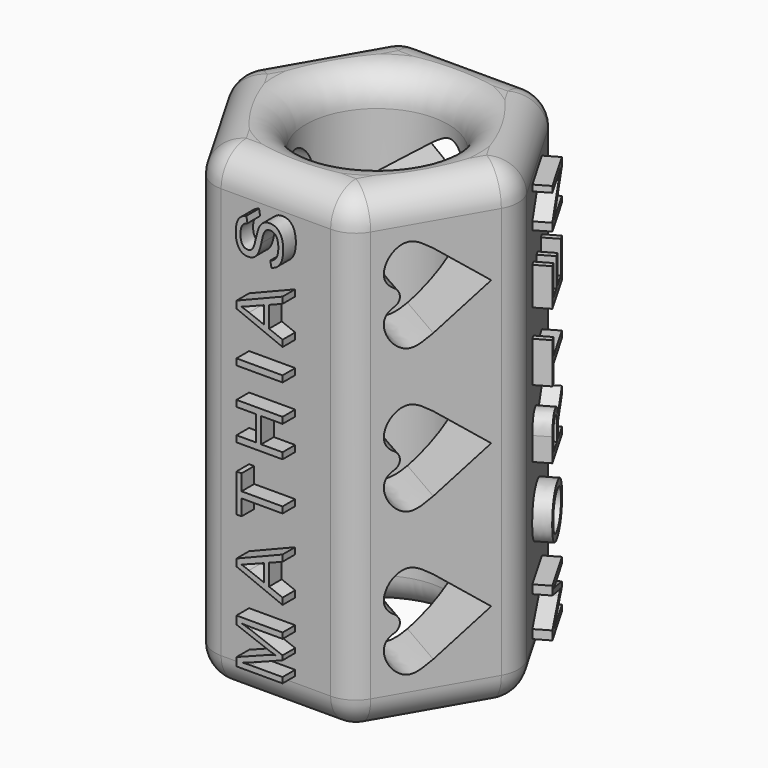
from build123d import *

# Parameters (mm, degrees)
F0_R          = 2.25
F1_DEPTH      = 15
F2_TEXT_SIZE  = 2.9915144542
F3_DEPTH      = 0.5
F4_TEXT_SIZE  = 2.2767698328
F5_DEPTH      = 0.5
F6_TEXT_SIZE  = 2.1189354387
F7_DEPTH      = 0.5
F9_DEPTH      = 5
F11_DEPTH     = 5
F13_DEPTH     = 5
F14_T1_DEPTH  = 9.6188021535
F14_T3_DEPTH  = 9.6188021535
F14_T5_DEPTH  = 9.6188021535
F14_T7_DEPTH  = 9.6188021535
F14_T9_DEPTH  = 9.6188021535
F15_T1_DEPTH  = 13
F15_T6_DEPTH  = 1
F15_T12_DEPTH = 1
F15_T18_DEPTH = 1
F15_T24_DEPTH = 1
F15_T30_DEPTH = 1
F15_T36_DEPTH = 1
F15_T42_DEPTH = 1
F15_T48_DEPTH = 1
F15_T54_DEPTH = 1
F15_T60_DEPTH = 1
F15_T66_DEPTH = 1
F15_T72_DEPTH = 1
F16_R         = 0.3


# Not quite as in the source:
# - a fillet or chamfer that OpenCascade refuses, or shapes differently, is made with other operations: its cross-section is extruded or revolved along the edge and cut away or added
# - Text() gives the source's letters only with a copy of the font that has no kerning and outlines rounded to 1/6400 em; it was checked with that copy


with BuildPart() as f1:
    # F0 (on Top) → F1 (new body)
    with BuildSketch(Plane.XY):
        Polygon((-2.3094010768, -4), (2.3094010768, -4), (4.6188021535, 0), (2.3094010768, 4), (-2.3094010768, 4), (-4.6188021535, 0), align=None)
        Circle(F0_R, mode=Mode.SUBTRACT)
    extrude(amount=F1_DEPTH)

    # F2 (on face) → F3 (join)
    with BuildSketch(Plane(origin=(-3.4641016151, 2, 0), x_dir=(-0.5, -0.8660254038, 0), z_dir=(-0.8660254038, 0.5, 0))):
        with Locations(Location((0.9215387268, 1), (0, 0, 90))):
            Text('M A R I A', F2_TEXT_SIZE, font='Arimo', text_align=(TextAlign.LEFT, TextAlign.BOTTOM))
    extrude(amount=F3_DEPTH)

    # F4 (on face) → F5 (join)
    with BuildSketch(Plane(origin=(3.4641016151, 2, 0), x_dir=(-0.5, 0.8660254038, 0), z_dir=(0.8660254038, 0.5, 0))):
        with Locations(Location((0.7773110224, 0.9308314361), (0, 0, 90))):
            Text('M O R T E N', F4_TEXT_SIZE, font='Arimo', text_align=(TextAlign.LEFT, TextAlign.BOTTOM))
    extrude(amount=F5_DEPTH)

    # F6 (on face) → F7 (join)
    with BuildSketch(Plane.XZ.offset(4)):
        with Locations(Location((0.6108914517, 1.017461665), (0, 0, 90))):
            Text('M A T H I A S', F6_TEXT_SIZE, font='Arimo', text_align=(TextAlign.LEFT, TextAlign.BOTTOM))
    extrude(amount=F7_DEPTH)

    # F8 (on face) → F9 (cut)
    with BuildSketch(Plane(origin=(-3.4641016151, -2, 0), x_dir=(0.5, -0.8660254038, 0), z_dir=(-0.8660254038, -0.5, 0))):
        with BuildLine():
            Line((0, 1.776238773), (1.5377772506, 2.9594601877))
            Line((1.5377772506, 2.9594601877), (0, 4.1426816024))
            add(Edge.make_bspline(
                [(0, 4.1426816024), (-0.2173509057, 4.2946153333), (-0.6310612999, 4.5838092683), (-1.2004435179, 4.1850955605), (-1.3756111709, 3.5968057921), (-1.1404542273, 3.2179649778), (-0.5606131931, 3.0412608869), (-0.1866981793, 2.9867018613), (0, 2.9594601877)],
                knots=[0, 0, 0, 0, 0.1874012518, 0.3567035782, 0.5239209237, 0.6616950004, 0.8310821306, 1, 1, 1, 1], degree=3))
            add(Edge.make_bspline(
                [(0, 1.776238773), (-0.2173509057, 1.6243050422), (-0.6310612999, 1.3351111071), (-1.2004435179, 1.7338248149), (-1.3756111709, 2.3221145833), (-1.1404542273, 2.7009553976), (-0.5606131931, 2.8776594885), (-0.1866981793, 2.9322185141), (0, 2.9594601877)],
                knots=[0, 0, 0, 0, 0.1874012518, 0.3567035782, 0.5239209237, 0.6616950004, 0.8310821306, 1, 1, 1, 1], degree=3))
        make_face()
        with BuildLine():
            Line((0, 6.3167785853), (1.5377772506, 7.5))
            Line((1.5377772506, 7.5), (0, 8.6832214147))
            add(Edge.make_bspline(
                [(0, 8.6832214147), (-0.2173509057, 8.8351551455), (-0.6310612999, 9.1243490806), (-1.2004435179, 8.7256353728), (-1.3756111709, 8.1373456044), (-1.1404542273, 7.7585047901), (-0.5606131931, 7.5818006992), (-0.1866981793, 7.5272416736), (0, 7.5)],
                knots=[0, 0, 0, 0, 0.1874012518, 0.3567035782, 0.5239209237, 0.6616950004, 0.8310821306, 1, 1, 1, 1], degree=3))
            add(Edge.make_bspline(
                [(0, 6.3167785853), (-0.2173509057, 6.1648448545), (-0.6310612999, 5.8756509194), (-1.2004435179, 6.2743646272), (-1.3756111709, 6.8626543956), (-1.1404542273, 7.2414952099), (-0.5606131931, 7.4181993008), (-0.1866981793, 7.4727583264), (0, 7.5)],
                knots=[0, 0, 0, 0, 0.1874012518, 0.3567035782, 0.5239209237, 0.6616950004, 0.8310821306, 1, 1, 1, 1], degree=3))
        make_face()
        with BuildLine():
            Line((0, 10.8573183976), (1.5377772506, 12.0405398123))
            Line((1.5377772506, 12.0405398123), (0, 13.223761227))
            add(Edge.make_bspline(
                [(0, 13.223761227), (-0.2173509057, 13.3756949578), (-0.6310612999, 13.6648888929), (-1.2004435179, 13.2661751851), (-1.3756111709, 12.6778854167), (-1.1404542273, 12.2990446024), (-0.5606131931, 12.1223405115), (-0.1866981793, 12.0677814859), (0, 12.0405398123)],
                knots=[0, 0, 0, 0, 0.1874012518, 0.3567035782, 0.5239209237, 0.6616950004, 0.8310821306, 1, 1, 1, 1], degree=3))
            add(Edge.make_bspline(
                [(0, 10.8573183976), (-0.2173509057, 10.7053846667), (-0.6310612999, 10.4161907317), (-1.2004435179, 10.8149044395), (-1.3756111709, 11.4031942079), (-1.1404542273, 11.7820350222), (-0.5606131931, 11.9587391131), (-0.1866981793, 12.0132981387), (0, 12.0405398123)],
                knots=[0, 0, 0, 0, 0.1874012518, 0.3567035782, 0.5239209237, 0.6616950004, 0.8310821306, 1, 1, 1, 1], degree=3))
        make_face()
    extrude(amount=-F9_DEPTH, mode=Mode.SUBTRACT)

    # F10 (on face) → F11 (cut)
    with BuildSketch(Plane(origin=(0, 4, 0), x_dir=(-1, 0, 0), z_dir=(0, 1, 0))):
        with BuildLine():
            Line((0.0039297288, 6.4260225961), (1.5417069794, 7.6092440108))
            Line((1.5417069794, 7.6092440108), (0.0039297288, 8.7924654255))
            add(Edge.make_bspline(
                [(0.0039297288, 8.7924654255), (-0.2134211769, 8.9443991563), (-0.6271315711, 9.2335930914), (-1.1965137892, 8.8348793835), (-1.3716814422, 8.2465896152), (-1.1365244985, 7.8677488009), (-0.5566834644, 7.69104471), (-0.1827684505, 7.6364856844), (0.0039297288, 7.6092440108)],
                knots=[0, 0, 0, 0, 0.1874012518, 0.3567035782, 0.5239209237, 0.6616950004, 0.8310821306, 1, 1, 1, 1], degree=3))
            add(Edge.make_bspline(
                [(0.0039297288, 6.4260225961), (-0.2134211769, 6.2740888652), (-0.6271315711, 5.9848949302), (-1.1965137892, 6.383608638), (-1.3716814422, 6.9718984064), (-1.1365244985, 7.3507392207), (-0.5566834644, 7.5274433116), (-0.1827684505, 7.5820023372), (0.0039297288, 7.6092440108)],
                knots=[0, 0, 0, 0, 0.1874012518, 0.3567035782, 0.5239209237, 0.6616950004, 0.8310821306, 1, 1, 1, 1], degree=3))
        make_face()
        with BuildLine():
            Line((0.0039297288, 10.9665624084), (1.5417069794, 12.1497838231))
            Line((1.5417069794, 12.1497838231), (0.0039297288, 13.3330052378))
            add(Edge.make_bspline(
                [(0.0039297288, 13.3330052378), (-0.2134211769, 13.4849389686), (-0.6271315711, 13.7741329037), (-1.1965137892, 13.3754191958), (-1.3716814422, 12.7871294275), (-1.1365244985, 12.4082886132), (-0.5566834644, 12.2315845223), (-0.1827684505, 12.1770254967), (0.0039297288, 12.1497838231)],
                knots=[0, 0, 0, 0, 0.1874012518, 0.3567035782, 0.5239209237, 0.6616950004, 0.8310821306, 1, 1, 1, 1], degree=3))
            add(Edge.make_bspline(
                [(0.0039297288, 10.9665624084), (-0.2134211769, 10.8146286775), (-0.6271315711, 10.5254347425), (-1.1965137892, 10.9241484503), (-1.3716814422, 11.5124382187), (-1.1365244985, 11.891279033), (-0.5566834644, 12.0679831239), (-0.1827684505, 12.1225421495), (0.0039297288, 12.1497838231)],
                knots=[0, 0, 0, 0, 0.1874012518, 0.3567035782, 0.5239209237, 0.6616950004, 0.8310821306, 1, 1, 1, 1], degree=3))
        make_face()
        with BuildLine():
            Line((0.0039297288, 1.8854827838), (1.5417069794, 3.0687041985))
            Line((1.5417069794, 3.0687041985), (0.0039297288, 4.2519256132))
            add(Edge.make_bspline(
                [(0.0039297288, 4.2519256132), (-0.2134211769, 4.403859344), (-0.6271315711, 4.6930532791), (-1.1965137892, 4.2943395713), (-1.3716814422, 3.7060498029), (-1.1365244985, 3.3272089886), (-0.5566834644, 3.1505048977), (-0.1827684505, 3.0959458721), (0.0039297288, 3.0687041985)],
                knots=[0, 0, 0, 0, 0.1874012518, 0.3567035782, 0.5239209237, 0.6616950004, 0.8310821306, 1, 1, 1, 1], degree=3))
            add(Edge.make_bspline(
                [(0.0039297288, 1.8854827838), (-0.2134211769, 1.7335490529), (-0.6271315711, 1.4443551179), (-1.1965137892, 1.8430688257), (-1.3716814422, 2.4313585941), (-1.1365244985, 2.8101994084), (-0.5566834644, 2.9869034993), (-0.1827684505, 3.0414625249), (0.0039297288, 3.0687041985)],
                knots=[0, 0, 0, 0, 0.1874012518, 0.3567035782, 0.5239209237, 0.6616950004, 0.8310821306, 1, 1, 1, 1], degree=3))
        make_face()
    extrude(amount=-F11_DEPTH, mode=Mode.SUBTRACT)

    # F12 (on face) → F13 (cut)
    with BuildSketch(Plane(origin=(3.4641016151, -2, 0), x_dir=(0.5, 0.8660254038, 0), z_dir=(0.8660254038, -0.5, 0))):
        with BuildLine():
            Line((-0.0730864861, 6.3305400545), (1.4646907645, 7.5137614692))
            Line((1.4646907645, 7.5137614692), (-0.0730864861, 8.6969828838))
            add(Edge.make_bspline(
                [(-0.0730864861, 8.6969828838), (-0.2904373917, 8.8489166147), (-0.704147786, 9.1381105498), (-1.273530004, 8.7393968419), (-1.448697657, 8.1511070736), (-1.2135407134, 7.7722662592), (-0.6336996792, 7.5955621684), (-0.2597846654, 7.5410031427), (-0.0730864861, 7.5137614692)],
                knots=[0, 0, 0, 0, 0.1874012518, 0.3567035782, 0.5239209237, 0.6616950004, 0.8310821306, 1, 1, 1, 1], degree=3))
            add(Edge.make_bspline(
                [(-0.0730864861, 6.3305400545), (-0.2904373917, 6.1786063236), (-0.704147786, 5.8894123886), (-1.273530004, 6.2881260964), (-1.448697657, 6.8764158648), (-1.2135407134, 7.2552566791), (-0.6336996792, 7.43196077), (-0.2597846654, 7.4865197956), (-0.0730864861, 7.5137614692)],
                knots=[0, 0, 0, 0, 0.1874012518, 0.3567035782, 0.5239209237, 0.6616950004, 0.8310821306, 1, 1, 1, 1], degree=3))
        make_face()
        with BuildLine():
            Line((-0.0730864861, 10.8710798668), (1.4646907645, 12.0543012815))
            Line((1.4646907645, 12.0543012815), (-0.0730864861, 13.2375226961))
            add(Edge.make_bspline(
                [(-0.0730864861, 13.2375226961), (-0.2904373917, 13.389456427), (-0.704147786, 13.678650362), (-1.273530004, 13.2799366542), (-1.448697657, 12.6916468859), (-1.2135407134, 12.3128060715), (-0.6336996792, 12.1361019807), (-0.2597846654, 12.081542955), (-0.0730864861, 12.0543012815)],
                knots=[0, 0, 0, 0, 0.1874012518, 0.3567035782, 0.5239209237, 0.6616950004, 0.8310821306, 1, 1, 1, 1], degree=3))
            add(Edge.make_bspline(
                [(-0.0730864861, 10.8710798668), (-0.2904373917, 10.7191461359), (-0.704147786, 10.4299522009), (-1.273530004, 10.8286659087), (-1.448697657, 11.4169556771), (-1.2135407134, 11.7957964914), (-0.6336996792, 11.9725005823), (-0.2597846654, 12.0270596079), (-0.0730864861, 12.0543012815)],
                knots=[0, 0, 0, 0, 0.1874012518, 0.3567035782, 0.5239209237, 0.6616950004, 0.8310821306, 1, 1, 1, 1], degree=3))
        make_face()
        with BuildLine():
            Line((-0.0730864861, 1.7900002422), (1.4646907645, 2.9732216569))
            Line((1.4646907645, 2.9732216569), (-0.0730864861, 4.1564430716))
            add(Edge.make_bspline(
                [(-0.0730864861, 4.1564430716), (-0.2904373917, 4.3083768024), (-0.704147786, 4.5975707375), (-1.273530004, 4.1988570296), (-1.448697657, 3.6105672613), (-1.2135407134, 3.2317264469), (-0.6336996792, 3.0550223561), (-0.2597846654, 3.0004633304), (-0.0730864861, 2.9732216569)],
                knots=[0, 0, 0, 0, 0.1874012518, 0.3567035782, 0.5239209237, 0.6616950004, 0.8310821306, 1, 1, 1, 1], degree=3))
            add(Edge.make_bspline(
                [(-0.0730864861, 1.7900002422), (-0.2904373917, 1.6380665113), (-0.704147786, 1.3488725763), (-1.273530004, 1.7475862841), (-1.448697657, 2.3358760525), (-1.2135407134, 2.7147168668), (-0.6336996792, 2.8914209577), (-0.2597846654, 2.9459799833), (-0.0730864861, 2.9732216569)],
                knots=[0, 0, 0, 0, 0.1874012518, 0.3567035782, 0.5239209237, 0.6616950004, 0.8310821306, 1, 1, 1, 1], degree=3))
        make_face()
    extrude(amount=-F13_DEPTH, mode=Mode.SUBTRACT)

    # F14: fillet of radius 1 on 14 edges, made by hand

    # F14_s2 → F14_t1 (cut)
    with BuildSketch(Plane.YZ.offset(-4.8094010768)):
        with BuildLine():
            ThreePointArc((-4, 14), (-3.7071067812, 14.7071067812), (-3, 15))
            Line((-3, 15), (-4, 15))
            Line((-4, 15), (-4, 14))
        make_face()
        with BuildLine():
            ThreePointArc((3, 15), (3.7071067812, 14.7071067812), (4, 14))
            Line((4, 14), (4, 15))
            Line((4, 15), (3, 15))
        make_face()
        with BuildLine():
            ThreePointArc((-4, 1), (-3.7071067812, 0.2928932188), (-3, 0))
            Line((-3, 0), (-4, 0))
            Line((-4, 0), (-4, 1))
        make_face()
        with BuildLine():
            ThreePointArc((3, 0), (3.7071067812, 0.2928932188), (4, 1))
            Line((4, 1), (4, 0))
            Line((4, 0), (3, 0))
        make_face()
    extrude(amount=F14_T1_DEPTH, mode=Mode.SUBTRACT)

    # F14_s4 → F14_t3 (cut)
    with BuildSketch(Plane(origin=(-2.4047005384, -4.1650635095, 0), x_dir=(0, 0, 1), z_dir=(0.5, 0.8660254038, 0))):
        with BuildLine():
            ThreePointArc((15, 3), (14.7071067812, 3.7071067812), (14, 4))
            Line((14, 4), (15, 4))
            Line((15, 4), (15, 3))
        make_face()
        with BuildLine():
            ThreePointArc((0, 3), (0.2928932188, 3.7071067812), (1, 4))
            Line((1, 4), (0, 4))
            Line((0, 4), (0, 3))
        make_face()
    extrude(amount=F14_T3_DEPTH, mode=Mode.SUBTRACT)

    # F14_s6 → F14_t5 (cut)
    with BuildSketch(Plane(origin=(2.4047005384, -4.1650635095, 0), x_dir=(0, 0, 1), z_dir=(-0.5, 0.8660254038, 0))):
        with BuildLine():
            ThreePointArc((15, 3), (14.7071067812, 3.7071067812), (14, 4))
            Line((14, 4), (15, 4))
            Line((15, 4), (15, 3))
        make_face()
        with BuildLine():
            ThreePointArc((0, 3), (0.2928932188, 3.7071067812), (1, 4))
            Line((1, 4), (0, 4))
            Line((0, 4), (0, 3))
        make_face()
    extrude(amount=F14_T5_DEPTH, mode=Mode.SUBTRACT)

    # F14_s8 → F14_t7 (cut)
    with BuildSketch(Plane(origin=(2.4047005384, 4.1650635095, 0), x_dir=(0, 0, 1), z_dir=(-0.5, -0.8660254038, 0))):
        with BuildLine():
            ThreePointArc((15, 3), (14.7071067812, 3.7071067812), (14, 4))
            Line((14, 4), (15, 4))
            Line((15, 4), (15, 3))
        make_face()
        with BuildLine():
            ThreePointArc((0, 3), (0.2928932188, 3.7071067812), (1, 4))
            Line((1, 4), (0, 4))
            Line((0, 4), (0, 3))
        make_face()
    extrude(amount=F14_T7_DEPTH, mode=Mode.SUBTRACT)

    # F14_s10 → F14_t9 (cut)
    with BuildSketch(Plane(origin=(-2.4047005384, 4.1650635095, 0), x_dir=(0, 0, 1), z_dir=(0.5, -0.8660254038, 0))):
        with BuildLine():
            ThreePointArc((14, 4), (14.7071067812, 3.7071067812), (15, 3))
            Line((15, 3), (15, 4))
            Line((15, 4), (14, 4))
        make_face()
        with BuildLine():
            ThreePointArc((1, 4), (0.2928932188, 3.7071067812), (0, 3))
            Line((0, 3), (0, 4))
            Line((0, 4), (1, 4))
        make_face()
    extrude(amount=F14_T9_DEPTH, mode=Mode.SUBTRACT)

    # F14_s11 → F14_t12 (revolve, cut)
    with BuildSketch(Plane.XZ):
        with BuildLine():
            ThreePointArc((3.25, 15), (2.5428932188, 14.7071067812), (2.25, 14))
            Line((2.25, 14), (2.25, 15))
            Line((2.25, 15), (3.25, 15))
        make_face()
    revolve(axis=Axis((0, 0, 15), (0, 0, 1)), mode=Mode.SUBTRACT)

    # F14_s13 → F14_t14 (revolve, cut)
    with BuildSketch(Plane.XZ):
        with BuildLine():
            ThreePointArc((3.25, 0), (2.5428932188, 0.2928932188), (2.25, 1))
            Line((2.25, 1), (2.25, 0))
            Line((2.25, 0), (3.25, 0))
        make_face()
    revolve(axis=Axis((0, 0, 0), (0, 0, 1)), mode=Mode.SUBTRACT)

    # F15: fillet of radius 1 on 6 edges, made by hand

    # F15_s2 → F15_t1 (cut)
    with BuildSketch(Plane.XY.offset(1)):
        with BuildLine():
            ThreePointArc((1.7320508076, -4), (2.2320508076, -3.8660254038), (2.5980762114, -3.5))
            Line((2.5980762114, -3.5), (2.3094010768, -4))
            Line((2.3094010768, -4), (1.7320508076, -4))
        make_face()
        with BuildLine():
            ThreePointArc((4.3301270189, -0.5), (4.4641016151, 0), (4.3301270189, 0.5))
            Line((4.3301270189, 0.5), (4.6188021535, 0))
            Line((4.6188021535, 0), (4.3301270189, -0.5))
        make_face()
        with BuildLine():
            ThreePointArc((2.5980762114, 3.5), (2.2320508076, 3.8660254038), (1.7320508076, 4))
            Line((1.7320508076, 4), (2.3094010768, 4))
            Line((2.3094010768, 4), (2.5980762114, 3.5))
        make_face()
        with BuildLine():
            ThreePointArc((-2.5980762114, 3.5), (-2.2320508076, 3.8660254038), (-1.7320508076, 4))
            Line((-1.7320508076, 4), (-2.3094010768, 4))
            Line((-2.3094010768, 4), (-2.5980762114, 3.5))
        make_face()
        with BuildLine():
            ThreePointArc((-4.3301270189, -0.5), (-4.4641016151, 0), (-4.3301270189, 0.5))
            Line((-4.3301270189, 0.5), (-4.6188021535, 0))
            Line((-4.6188021535, 0), (-4.3301270189, -0.5))
        make_face()
        with BuildLine():
            ThreePointArc((-1.7320508076, -4), (-2.2320508076, -3.8660254038), (-2.5980762114, -3.5))
            Line((-2.5980762114, -3.5), (-2.3094010768, -4))
            Line((-2.3094010768, -4), (-1.7320508076, -4))
        make_face()
    extrude(amount=F15_T1_DEPTH, mode=Mode.SUBTRACT)


with BuildPart() as f15_tool4:
    # F15_s5 → F15_t6 (new body)
    with BuildSketch(Plane.XY.offset(1)):
        Polygon((-1.7320508076, -3), (-1.7320508076, -4), (-2.3094010768, -4), (-2.5980762114, -3.5), align=None)
    extrude(amount=-F15_T6_DEPTH)

    # F15_s7 → F15_t8 (revolve, cut)
    with BuildSketch(Plane(origin=(-1.7320508076, -3, 1), x_dir=(0.5, 0.8660254038, 0), z_dir=(-0.8660254038, 0.5, 0))):
        with BuildLine():
            ThreePointArc((0, -1), (1, 0), (0, 1))
            Line((0, 1), (0, -1))
        make_face()
    revolve(axis=Axis((-1.7320508076, -3, 1), (0, 0, -1)), mode=Mode.SUBTRACT)


with BuildPart() as f1_1:
    add(f1.part)

    # F15_t3: cut F15_tool4
    add(f15_tool4.part, mode=Mode.SUBTRACT)


with BuildPart() as f15_tool10:
    # F15_s11 → F15_t12 (new body)
    with BuildSketch(Plane.XY.offset(14)):
        Polygon((-1.7320508076, -3), (-1.7320508076, -4), (-2.3094010768, -4), (-2.5980762114, -3.5), align=None)
    extrude(amount=F15_T12_DEPTH)

    # F15_s13 → F15_t14 (revolve, cut)
    with BuildSketch(Plane(origin=(-1.7320508076, -3, 14), x_dir=(0.5, 0.8660254038, 0), z_dir=(0.8660254038, -0.5, 0))):
        with BuildLine():
            ThreePointArc((0, -1), (1, 0), (0, 1))
            Line((0, 1), (0, -1))
        make_face()
    revolve(axis=Axis((-1.7320508076, -3, 14), (0, 0, 1)), mode=Mode.SUBTRACT)


with BuildPart() as f1_2:
    add(f1_1.part)

    # F15_t9: cut F15_tool10
    add(f15_tool10.part, mode=Mode.SUBTRACT)


with BuildPart() as f15_tool16:
    # F15_s17 → F15_t18 (new body)
    with BuildSketch(Plane.XY.offset(1)):
        Polygon((-3.4641016151, 0), (-4.3301270189, -0.5), (-4.6188021535, 0), (-4.3301270189, 0.5), align=None)
    extrude(amount=-F15_T18_DEPTH)

    # F15_s19 → F15_t20 (revolve, cut)
    with BuildSketch(Plane(origin=(-3.4641016151, 0, 1), x_dir=(1, 0, 0), z_dir=(0, 1, 0))):
        with BuildLine():
            ThreePointArc((0, -1), (1, 0), (0, 1))
            Line((0, 1), (0, -1))
        make_face()
    revolve(axis=Axis((-3.4641016151, 0, 1), (0, 0, -1)), mode=Mode.SUBTRACT)


with BuildPart() as f1_3:
    add(f1_2.part)

    # F15_t15: cut F15_tool16
    add(f15_tool16.part, mode=Mode.SUBTRACT)


with BuildPart() as f15_tool22:
    # F15_s23 → F15_t24 (new body)
    with BuildSketch(Plane.XY.offset(14)):
        Polygon((-3.4641016151, 0), (-4.3301270189, -0.5), (-4.6188021535, 0), (-4.3301270189, 0.5), align=None)
    extrude(amount=F15_T24_DEPTH)

    # F15_s25 → F15_t26 (revolve, cut)
    with BuildSketch(Plane(origin=(-3.4641016151, 0, 14), x_dir=(1, 0, 0), z_dir=(0, -1, 0))):
        with BuildLine():
            ThreePointArc((0, -1), (1, 0), (0, 1))
            Line((0, 1), (0, -1))
        make_face()
    revolve(axis=Axis((-3.4641016151, 0, 14), (0, 0, 1)), mode=Mode.SUBTRACT)


with BuildPart() as f1_4:
    add(f1_3.part)

    # F15_t21: cut F15_tool22
    add(f15_tool22.part, mode=Mode.SUBTRACT)


with BuildPart() as f15_tool28:
    # F15_s29 → F15_t30 (new body)
    with BuildSketch(Plane.XY.offset(1)):
        Polygon((-1.7320508076, 3), (-2.5980762114, 3.5), (-2.3094010768, 4), (-1.7320508076, 4), align=None)
    extrude(amount=-F15_T30_DEPTH)

    # F15_s31 → F15_t32 (revolve, cut)
    with BuildSketch(Plane(origin=(-1.7320508076, 3, 1), x_dir=(0.5, -0.8660254038, 0), z_dir=(0.8660254038, 0.5, 0))):
        with BuildLine():
            ThreePointArc((0, -1), (1, 0), (0, 1))
            Line((0, 1), (0, -1))
        make_face()
    revolve(axis=Axis((-1.7320508076, 3, 1), (0, 0, -1)), mode=Mode.SUBTRACT)


with BuildPart() as f1_5:
    add(f1_4.part)

    # F15_t27: cut F15_tool28
    add(f15_tool28.part, mode=Mode.SUBTRACT)


with BuildPart() as f15_tool34:
    # F15_s35 → F15_t36 (new body)
    with BuildSketch(Plane.XY.offset(14)):
        Polygon((-1.7320508076, 3), (-2.5980762114, 3.5), (-2.3094010768, 4), (-1.7320508076, 4), align=None)
    extrude(amount=F15_T36_DEPTH)

    # F15_s37 → F15_t38 (revolve, cut)
    with BuildSketch(Plane(origin=(-1.7320508076, 3, 14), x_dir=(0.5, -0.8660254038, 0), z_dir=(-0.8660254038, -0.5, 0))):
        with BuildLine():
            ThreePointArc((0, -1), (1, 0), (0, 1))
            Line((0, 1), (0, -1))
        make_face()
    revolve(axis=Axis((-1.7320508076, 3, 14), (0, 0, 1)), mode=Mode.SUBTRACT)


with BuildPart() as f1_6:
    add(f1_5.part)

    # F15_t33: cut F15_tool34
    add(f15_tool34.part, mode=Mode.SUBTRACT)


with BuildPart() as f15_tool40:
    # F15_s41 → F15_t42 (new body)
    with BuildSketch(Plane.XY.offset(1)):
        Polygon((1.7320508076, 3), (2.5980762114, 3.5), (2.3094010768, 4), (1.7320508076, 4), align=None)
    extrude(amount=-F15_T42_DEPTH)

    # F15_s43 → F15_t44 (revolve, cut)
    with BuildSketch(Plane(origin=(1.7320508076, 3, 1), x_dir=(-0.5, -0.8660254038, 0), z_dir=(0.8660254038, -0.5, 0))):
        with BuildLine():
            ThreePointArc((0, -1), (1, 0), (0, 1))
            Line((0, 1), (0, -1))
        make_face()
    revolve(axis=Axis((1.7320508076, 3, 1), (0, 0, -1)), mode=Mode.SUBTRACT)


with BuildPart() as f1_7:
    add(f1_6.part)

    # F15_t39: cut F15_tool40
    add(f15_tool40.part, mode=Mode.SUBTRACT)


with BuildPart() as f15_tool46:
    # F15_s47 → F15_t48 (new body)
    with BuildSketch(Plane.XY.offset(14)):
        Polygon((1.7320508076, 3), (2.5980762114, 3.5), (2.3094010768, 4), (1.7320508076, 4), align=None)
    extrude(amount=F15_T48_DEPTH)

    # F15_s49 → F15_t50 (revolve, cut)
    with BuildSketch(Plane(origin=(1.7320508076, 3, 14), x_dir=(-0.5, -0.8660254038, 0), z_dir=(-0.8660254038, 0.5, 0))):
        with BuildLine():
            ThreePointArc((0, -1), (1, 0), (0, 1))
            Line((0, 1), (0, -1))
        make_face()
    revolve(axis=Axis((1.7320508076, 3, 14), (0, 0, 1)), mode=Mode.SUBTRACT)


with BuildPart() as f1_8:
    add(f1_7.part)

    # F15_t45: cut F15_tool46
    add(f15_tool46.part, mode=Mode.SUBTRACT)


with BuildPart() as f15_tool52:
    # F15_s53 → F15_t54 (new body)
    with BuildSketch(Plane.XY.offset(1)):
        Polygon((3.4641016151, 0), (4.3301270189, -0.5), (4.6188021535, 0), (4.3301270189, 0.5), align=None)
    extrude(amount=-F15_T54_DEPTH)

    # F15_s55 → F15_t56 (revolve, cut)
    with BuildSketch(Plane(origin=(3.4641016151, 0, 1), x_dir=(-1, 0, 0), z_dir=(0, -1, 0))):
        with BuildLine():
            ThreePointArc((0, -1), (1, 0), (0, 1))
            Line((0, 1), (0, -1))
        make_face()
    revolve(axis=Axis((3.4641016151, 0, 1), (0, 0, -1)), mode=Mode.SUBTRACT)


with BuildPart() as f1_9:
    add(f1_8.part)

    # F15_t51: cut F15_tool52
    add(f15_tool52.part, mode=Mode.SUBTRACT)


with BuildPart() as f15_tool58:
    # F15_s59 → F15_t60 (new body)
    with BuildSketch(Plane.XY.offset(14)):
        Polygon((3.4641016151, 0), (4.3301270189, -0.5), (4.6188021535, 0), (4.3301270189, 0.5), align=None)
    extrude(amount=F15_T60_DEPTH)

    # F15_s61 → F15_t62 (revolve, cut)
    with BuildSketch(Plane(origin=(3.4641016151, 0, 14), x_dir=(-1, 0, 0), z_dir=(0, 1, 0))):
        with BuildLine():
            ThreePointArc((0, -1), (1, 0), (0, 1))
            Line((0, 1), (0, -1))
        make_face()
    revolve(axis=Axis((3.4641016151, 0, 14), (0, 0, 1)), mode=Mode.SUBTRACT)


with BuildPart() as f1_10:
    add(f1_9.part)

    # F15_t57: cut F15_tool58
    add(f15_tool58.part, mode=Mode.SUBTRACT)


with BuildPart() as f15_tool64:
    # F15_s65 → F15_t66 (new body)
    with BuildSketch(Plane.XY.offset(1)):
        Polygon((1.7320508076, -3), (1.7320508076, -4), (2.3094010768, -4), (2.5980762114, -3.5), align=None)
    extrude(amount=-F15_T66_DEPTH)

    # F15_s67 → F15_t68 (revolve, cut)
    with BuildSketch(Plane(origin=(1.7320508076, -3, 1), x_dir=(-0.5, 0.8660254038, 0), z_dir=(-0.8660254038, -0.5, 0))):
        with BuildLine():
            ThreePointArc((0, -1), (1, 0), (0, 1))
            Line((0, 1), (0, -1))
        make_face()
    revolve(axis=Axis((1.7320508076, -3, 1), (0, 0, -1)), mode=Mode.SUBTRACT)


with BuildPart() as f1_11:
    add(f1_10.part)

    # F15_t63: cut F15_tool64
    add(f15_tool64.part, mode=Mode.SUBTRACT)


with BuildPart() as f15_tool70:
    # F15_s71 → F15_t72 (new body)
    with BuildSketch(Plane.XY.offset(14)):
        Polygon((1.7320508076, -3), (1.7320508076, -4), (2.3094010768, -4), (2.5980762114, -3.5), align=None)
    extrude(amount=F15_T72_DEPTH)

    # F15_s73 → F15_t74 (revolve, cut)
    with BuildSketch(Plane(origin=(1.7320508076, -3, 14), x_dir=(-0.5, 0.8660254038, 0), z_dir=(0.8660254038, 0.5, 0))):
        with BuildLine():
            ThreePointArc((0, -1), (1, 0), (0, 1))
            Line((0, 1), (0, -1))
        make_face()
    revolve(axis=Axis((1.7320508076, -3, 14), (0, 0, 1)), mode=Mode.SUBTRACT)


with BuildPart() as f1_12:
    add(f1_11.part)

    # F15_t69: cut F15_tool70
    add(f15_tool70.part, mode=Mode.SUBTRACT)

    # F16
    f16_edges = [f1_12.edges().sort_by_distance(p)[0] for p in [
        (-2.706329, -1.5625, 12.04054),
        (-2.706329, -1.5625, 7.5),
        (-2.706329, -1.5625, 2.95946),
        (-0.00393, 3.124998, 3.068704),
        (-0.00393, 3.124998, 7.609244),
        (-0.00393, 3.124998, 12.149784),
        (2.669272, -1.625498, 2.973222),
        (2.669272, -1.625498, 7.513761),
        (2.669272, -1.625498, 12.054301),
    ]]
    fillet(f16_edges, radius=F16_R)


solid = f1_12.part
